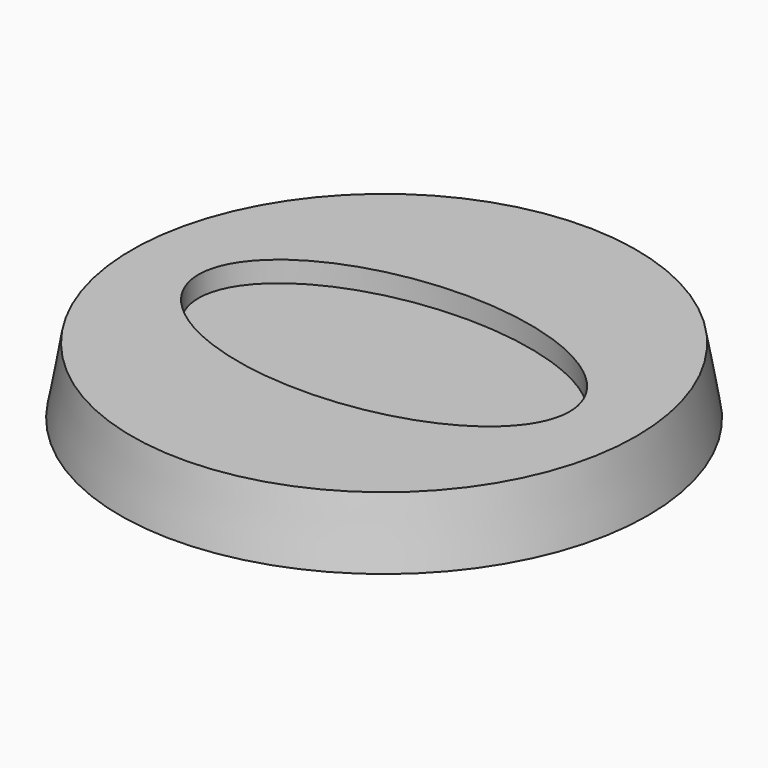
from build123d import *

# Parameters (mm, degrees)
F0_R     = 20
F1_DEPTH = 5
F2_SIZE2 = 0.881625
F2_SIZE  = 4.99999
F4_DEPTH = 1.5748


# Not quite as in the source:
# - a fillet or chamfer is up to 0.001 mm smaller than in the source, because OpenCascade refuses the exact size


with BuildPart() as f1:
    # F0 (on Top) → F1 (new body)
    with BuildSketch(Plane.XY):
        Circle(F0_R)
    extrude(amount=-F1_DEPTH)

    # F2 (size 5 and 0.8816349035 in the source; OpenCascade refuses exactly that, so slightly less here)
    f2_edges = [f1.edges().sort_by_distance(p)[0] for p in [
        (-20, 0, 0),
    ]]
    f2_side = f1.faces().sort_by_distance((-20, 0, -2.5))[0]
    chamfer(f2_edges, length=F2_SIZE, length2=F2_SIZE2, reference=f2_side)

    # F3 (on face) → F4 (cut)
    with BuildSketch(Plane.XY):
        with BuildLine():
            add(Edge.make_bspline(
                [(14.0589, 0), (14.0589, 13.5281828325), (-7.02945, 6.7640914163), (-28.1178, 0), (-7.02945, -6.7640914163), (14.0589, -13.5281828325), (14.0589, 0)],
                knots=[0, 0, 0, 2.0943951024, 2.0943951024, 4.1887902048, 4.1887902048, 6.2831853072, 6.2831853072, 6.2831853072], degree=2, weights=[1, 0.5, 1, 0.5, 1, 0.5, 1]))
        make_face()
    extrude(amount=-F4_DEPTH, mode=Mode.SUBTRACT)


solid = f1.part
